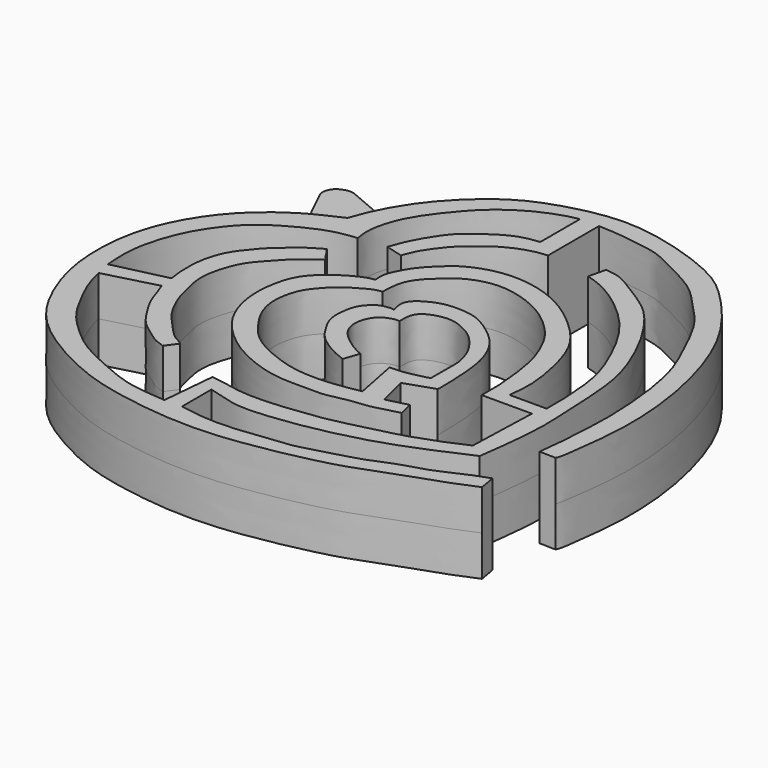
from build123d import *

# Parameters (mm, degrees)
F1_DEPTH    = 3.5
F3_DEPTH    = 2.5
F4_T1_DEPTH = 9.423215052
F4_T3_DEPTH = 7.2035331062
F4_T5_DEPTH = 6.3861082138
F6_R        = 1.3203003793
F7_DEPTH    = 5


# Not quite as in the source:
# - a fillet or chamfer that OpenCascade refuses, or shapes differently, is made with other operations: its cross-section is extruded or revolved along the edge and cut away or added
# - the dataset's text gives a spline's control points without its knots; the knots are read off the source's solid


with BuildPart() as f1:
    # F0 (on Top) → F1 (new body, symmetric)
    with BuildSketch(Plane.XY):
        with BuildLine():
            add(Edge.make_bspline(
                [(62.0494894683, 22.5223191082), (61.5763515234, 22.534451137), (61.1032135785, 22.5465831657), (60.6300756335, 22.5587151945)],
                knots=[0, 0, 0, 0, 1.4198803856, 1.4198803856, 1.4198803856, 1.4198803856], degree=3))
            add(Edge.make_bspline(
                [(29.0716737509, 41.1939695477), (29.306027893, 41.857310813), (29.8115589063, 43.2882259688), (31.339767814, 45.8344011789), (33.0379336105, 47.8185700655), (35.9160335187, 50.4486482505), (40.2057484134, 52.0426798575), (45.48861495, 52.9328004198), (52.9165185764, 50.5280179099), (55.6796708405, 48.398356233), (59.724609742, 43.8025024951), (61.9112576233, 37.8696812405), (62.8091572498, 32.726443865), (62.9266276354, 28.2018625321), (62.4240936499, 24.4927107006), (62.2361245052, 22.9214412082), (62.0494894683, 22.5223191082)],
                knots=[0, 0, 0, 0, 0.0521380391, 0.111927968, 0.1689619765, 0.2371588921, 0.3113537891, 0.3933259358, 0.4892077049, 0.5553764335, 0.6402636071, 0.729148712, 0.8091940033, 0.8840304935, 0.9524124, 1, 1, 1, 1], degree=3))
            add(Edge.make_bspline(
                [(60.8482062817, 16.0528682172), (60.4288818862, 15.8716763746), (59.534784142, 15.4853386593), (57.7264506978, 14.7998216857), (55.8708508075, 14.2034203061), (52.630731068, 12.9646220618), (50.9585172951, 12.4005941246), (47.9810616659, 11.6593155695), (45.2557239075, 11.174386798), (42.1471963462, 10.6964826332), (38.5794281807, 10.6237297735), (35.038597522, 10.9933372199), (30.8346536369, 11.7868657529), (27.2082918083, 13.3540305822), (23.6378704785, 15.5218973851), (21.3228934365, 17.9769063359), (19.6730407733, 21.3203975306), (18.6287885283, 25.130340922), (18.7791180909, 31.25108759), (22.1258241288, 36.9758945902), (26.2799285315, 39.9800364052), (27.8457582196, 40.6097996518), (29.0716737509, 41.1939695477)],
                knots=[0, 0, 0, 0, 0.0323172073, 0.0693227416, 0.1082559513, 0.158008347, 0.1950607871, 0.2415647298, 0.2872565248, 0.3350937464, 0.3860886927, 0.4374690356, 0.4931770933, 0.5474283537, 0.602365058, 0.6518805178, 0.7032339004, 0.7568993464, 0.8230773105, 0.8928533254, 0.9519441527, 1, 1, 1, 1], degree=3))
            add(Edge.make_bspline(
                [(60.5880208313, 17.5061523914), (60.6747493148, 17.0217243334), (60.7614777982, 16.5372962753), (60.8482062817, 16.0528682172)],
                knots=[0, 0, 0, 0, 1.4763913301, 1.4763913301, 1.4763913301, 1.4763913301], degree=3))
            add(Edge.make_bspline(
                [(37.5935249031, 12.5934553022), (38.0452848145, 12.531038319), (39.3071128132, 12.2668629621), (42.2147455771, 12.1754331807), (44.8674374333, 12.6506329659), (46.9396252013, 12.6974842254), (49.4646264533, 13.5274050404), (51.9887441448, 14.1045960088), (54.493210959, 15.2813445301), (56.3991158532, 15.6585487305), (59.124650253, 17.0151377844), (59.7854045823, 17.2054630189), (60.5880208313, 17.5061523914)],
                knots=[0, 0, 0, 0, 0.0839677582, 0.1958350575, 0.3028773071, 0.3959940813, 0.5007707763, 0.6070837185, 0.7133171176, 0.8066213923, 0.9144743817, 1, 1, 1, 1], degree=3))
            add(Edge.make_bspline(
                [(37.5935249031, 15.7923810184), (37.5935249031, 14.7863343979), (37.5935249031, 13.5995019227), (37.5935249031, 12.5934553022)],
                knots=[0, 0, 0, 0, 3.1989257162, 3.1989257162, 3.1989257162, 3.1989257162], degree=3))
            add(Edge.make_bspline(
                [(57.8698590398, 19.5260569453), (57.2722614614, 19.2518359716), (55.9374419677, 18.6547629093), (52.8317063751, 17.3486047041), (49.8839991865, 16.3833590419), (46.0118602733, 15.4908640908), (42.551168035, 15.058897568), (40.0725237694, 14.9739274299), (38.4607709731, 15.5945353022), (37.5935249031, 15.7923810184)],
                knots=[0, 0, 0, 0, 0.1197639567, 0.270468062, 0.4182518209, 0.5834884644, 0.7385810257, 0.8671389586, 1, 1, 1, 1], degree=3))
            add(Edge.make_bspline(
                [(47.4926754832, 46.1788736284), (47.927789971, 46.1352208019), (48.8780404031, 46.0398870027), (50.4485854452, 45.005540302), (52.793619445, 43.6144483568), (54.3147090185, 41.8964903618), (55.7547999729, 39.6954989953), (56.982321959, 37.1233650238), (57.9331963192, 34.4453501838), (58.2647103385, 31.2739474412), (58.3992190946, 27.6715420395), (58.5145376309, 25.6548387921), (58.3120615211, 22.7856589167), (58.0217878255, 20.6459678244), (57.8698590398, 19.5260569453)],
                knots=[0, 0, 0, 0, 0.0597690308, 0.1305301224, 0.2161422502, 0.2947520123, 0.3783962884, 0.4660421153, 0.5528551466, 0.6465286275, 0.7443886958, 0.8183602325, 0.9049300376, 1, 1, 1, 1], degree=3))
            add(Edge.make_bspline(
                [(47.1493708197, 44.6869616846), (47.2638057075, 45.1842656659), (47.3782405954, 45.6815696471), (47.4926754832, 46.1788736284)],
                knots=[0, 0, 0, 0, 1.5309014795, 1.5309014795, 1.5309014795, 1.5309014795], degree=3))
            add(Edge.make_bspline(
                [(57.0660457015, 27.7780741453), (57.0828094684, 28.3480911337), (57.0833657213, 29.4686732532), (56.9658779649, 31.452071832), (56.6597337165, 33.9116675307), (55.5444065948, 36.7282621966), (53.6693378682, 40.3548979754), (50.6815931716, 43.0058324291), (48.6285551485, 44.2222707419), (47.6501277942, 44.5268467146), (47.1493708197, 44.6869616846)],
                knots=[0, 0, 0, 0, 0.1014033342, 0.2110947118, 0.3333142833, 0.4693488673, 0.6282984434, 0.7850184408, 0.9039004269, 1, 1, 1, 1], degree=3))
            add(Edge.make_bspline(
                [(53.8438558578, 27.7780741453), (54.9179191391, 27.7780741453), (55.9919824203, 27.7780741453), (57.0660457015, 27.7780741453)],
                knots=[0, 0, 0, 0, 3.2221898437, 3.2221898437, 3.2221898437, 3.2221898437], degree=3))
            add(Edge.make_bspline(
                [(36.206882447, 35.2931544185), (36.1764845234, 35.5885803582), (36.1091925015, 36.2385932325), (36.6806068453, 37.4538685554), (37.3234322074, 38.5065184037), (38.5682458967, 39.7628057228), (39.7512814872, 40.7306689733), (42.5740597709, 41.7085320293), (45.9900359962, 41.2527105843), (48.8118848265, 39.8512735993), (51.2771955701, 37.6919484665), (52.6516823052, 35.8494727467), (53.4784180909, 33.5058638977), (53.9772231874, 30.8429033195), (54.0206694547, 29.2081760616), (53.9057321855, 28.3065811845), (53.8438558578, 27.7780741453)],
                knots=[0, 0, 0, 0, 0.0478150567, 0.1043645776, 0.1606219176, 0.225642618, 0.2873527464, 0.3715879872, 0.4636992782, 0.552438077, 0.6418664152, 0.7167824888, 0.7952255164, 0.8774223597, 0.9403869977, 1, 1, 1, 1], degree=3))
            add(Edge.make_bspline(
                [(49.791354686, 21.1576391011), (49.3382530631, 21.0376215345), (48.4902822396, 20.8130148085), (47.4767508433, 20.5043809637), (45.7231368878, 20.4183214673), (43.9634570973, 19.9068264066), (42.4944829734, 20.0241891308), (39.8604343147, 19.887922666), (37.1297080189, 20.7597202692), (35.0182532448, 21.8681586876), (32.9047601837, 23.6604882614), (31.6103804887, 25.6766069916), (30.9739740641, 28.0749194036), (31.1244725286, 30.4733894793), (31.7519799581, 32.5781705802), (33.5391654159, 34.172439048), (35.1990013305, 35.0808547127), (35.8615062461, 35.257202768), (36.206882447, 35.2931544185)],
                knots=[0, 0, 0, 0, 0.0512751396, 0.0967288377, 0.1552682074, 0.2149058996, 0.2683746399, 0.3397682684, 0.4148452727, 0.4835069411, 0.5564865603, 0.6248731942, 0.6939737689, 0.7623566152, 0.8270847949, 0.8952845577, 0.9556608186, 1, 1, 1, 1], degree=3))
            add(Edge.make_bspline(
                [(49.4943931699, 22.4225744605), (49.5933803419, 22.0009293407), (49.692367514, 21.5792842209), (49.791354686, 21.1576391011)],
                knots=[0, 0, 0, 0, 1.2993258273, 1.2993258273, 1.2993258273, 1.2993258273], degree=3))
            add(Edge.make_bspline(
                [(47.6537831128, 21.9598766416), (48.2673197985, 22.1141092479), (48.8808564842, 22.2683418542), (49.4943931699, 22.4225744605)],
                knots=[0, 0, 0, 0, 1.8978763537, 1.8978763537, 1.8978763537, 1.8978763537], degree=3))
            add(Edge.make_bspline(
                [(46.9948574901, 24.5558936149), (47.2144993643, 23.6905546238), (47.4341412385, 22.8252156327), (47.6537831128, 21.9598766416)],
                knots=[0, 0, 0, 0, 2.6783366296, 2.6783366296, 2.6783366296, 2.6783366296], degree=3))
            add(Edge.make_bspline(
                [(49.4943931699, 25.4038851708), (48.6612146099, 25.1212213188), (47.82803605, 24.8385574669), (46.9948574901, 24.5558936149)],
                knots=[0, 0, 0, 0, 2.6394636375, 2.6394636375, 2.6394636375, 2.6394636375], degree=3))
            add(Edge.make_bspline(
                [(39.9363972247, 32.6340422034), (39.8842838138, 32.8398562354), (39.7825802868, 33.2412074209), (39.7317090705, 33.8407763364), (40.1424327532, 34.4939511839), (40.9435667079, 34.98708908), (41.8689153893, 35.4022832836), (43.0578273832, 35.5288732917), (44.5042341477, 35.4172964468), (45.7031414177, 34.9277042276), (47.4978658208, 33.6142505705), (48.5069398345, 32.3164872915), (49.1750692015, 30.6332309556), (49.4127095767, 28.8730099925), (49.4897749365, 27.47010552), (49.5663415678, 25.7261840891), (49.5163608933, 25.5028841557), (49.4943931699, 25.4038851708)],
                knots=[0, 0, 0, 0, 0.0486624325, 0.0951159794, 0.1471567147, 0.20648322, 0.2679859547, 0.3350675936, 0.4079143723, 0.4781740436, 0.5686991634, 0.6479717232, 0.7297791406, 0.8106862151, 0.886747396, 0.9656619823, 1, 1, 1, 1], degree=3))
            add(Edge.make_bspline(
                [(41.731480509, 24.8407628387), (41.440631405, 24.9485887841), (40.8168018985, 25.1798651314), (39.7916131994, 25.7534846132), (38.7559420202, 26.5272756625), (38.0982481114, 27.4898951264), (37.2875541922, 28.8560847254), (37.3574485466, 30.3452179464), (37.6091145936, 31.571109546), (38.568811942, 32.5305731387), (39.2786992519, 32.6748706607), (39.7982324544, 32.7072710049), (39.9363972247, 32.6340422034)],
                knots=[0, 0, 0, 0, 0.0923950748, 0.1949164593, 0.3010659305, 0.4031182199, 0.5202614288, 0.6339443109, 0.739345279, 0.8450787721, 0.9263091339, 1, 1, 1, 1], degree=3))
            add(Edge.make_bspline(
                [(42.1944595873, 26.199799031), (42.0401332279, 25.7467869669), (41.8858068685, 25.2937749028), (41.731480509, 24.8407628387)],
                knots=[0, 0, 0, 0, 1.4357329135, 1.4357329135, 1.4357329135, 1.4357329135], degree=3))
            add(Edge.make_bspline(
                [(41.2784581907, 31.5763664872), (41.1436027927, 31.5858341266), (40.8403638146, 31.6097808209), (40.2362607189, 31.4043893185), (39.5927274842, 30.9978187711), (39.1784076019, 30.1464339224), (39.0659228719, 29.4295308466), (39.2309271665, 28.4702577556), (39.979528122, 27.528420715), (41.1981351902, 26.6654285399), (41.6937363632, 26.4125064221), (42.0679750848, 26.2360667755), (42.1944595873, 26.199799031)],
                knots=[0, 0, 0, 0, 0.0735226239, 0.1624191671, 0.2605026822, 0.3681233171, 0.4640931201, 0.5716419619, 0.6967882033, 0.8336292207, 0.9199382159, 1, 1, 1, 1], degree=3))
            add(Edge.make_bspline(
                [(48.1486208737, 26.3907369226), (48.1407468106, 26.8014264215), (48.1249530554, 28.1574826059), (48.2288835515, 29.260214228), (47.8216074376, 30.7540843594), (47.1971116739, 31.7848959678), (46.435927977, 32.6753941876), (45.7728156443, 33.1898699892), (44.5756440395, 33.8070333041), (43.4669023743, 33.9744272395), (42.0250272432, 33.6085927619), (41.2430052697, 32.8206115327), (41.2670391516, 32.0012648354), (41.2784581907, 31.5763664872)],
                knots=[0, 0, 0, 0, 0.1067685372, 0.1965667749, 0.2958638337, 0.3871372355, 0.4739417602, 0.549517036, 0.6427533045, 0.7302902948, 0.828194732, 0.9103637064, 1, 1, 1, 1], degree=3))
            add(Edge.make_bspline(
                [(44.9851080775, 25.8539021015), (45.4219860375, 25.8806252604), (46.2626284099, 25.8809088613), (47.208258913, 26.1637437155), (47.8616882143, 26.2615828811), (48.1486208737, 26.3907369226)],
                knots=[0, 0, 0, 0, 0.3648118806, 0.6850183006, 1, 1, 1, 1], degree=3))
            add(Edge.make_bspline(
                [(45.7483939826, 21.9598766416), (45.4939653476, 23.2578851283), (45.2395367126, 24.5558936149), (44.9851080775, 25.8539021015)],
                knots=[0, 0, 0, 0, 3.9681279787, 3.9681279787, 3.9681279787, 3.9681279787], degree=3))
            add(Edge.make_bspline(
                [(37.6781485975, 34.2296846211), (37.4404118501, 34.1936868052), (36.9248820688, 34.1220552019), (36.0572276042, 33.5790584889), (34.969351795, 33.007191617), (33.7116272309, 31.6576174543), (33.0250916628, 30.6155309796), (32.5469725534, 28.3648756243), (33.292716879, 26.3648713305), (34.1485984224, 25.1332402542), (35.0683346813, 23.9369652337), (36.4140307347, 22.972945278), (38.1110135143, 22.2170279083), (40.252083112, 21.514821624), (43.1220565262, 21.487846839), (44.8876694045, 21.8039903534), (45.7483939826, 21.9598766416)],
                knots=[0, 0, 0, 0, 0.0470759388, 0.1014443874, 0.162981057, 0.2361593674, 0.2979693267, 0.3790337951, 0.4585299897, 0.5253581662, 0.5918114662, 0.6616615194, 0.735923773, 0.8179351352, 0.9103719411, 1, 1, 1, 1], degree=3))
            add(Edge.make_bspline(
                [(52.3898104827, 26.5814382583), (52.4009236356, 27.1473973257), (52.422608099, 28.3284507078), (52.2339233546, 30.355819257), (51.8418938845, 33.0599256238), (50.7376318904, 35.5392708539), (49.6186905356, 36.9373328644), (47.9253669377, 38.4697088862), (45.4552778952, 39.6147669279), (42.8546664852, 39.989725932), (40.6509516266, 39.1817195979), (39.3514751131, 38.0710048359), (37.7393561929, 36.4275672316), (37.6985092177, 34.9608070194), (37.6781485975, 34.2296846211)],
                knots=[0, 0, 0, 0, 0.07336606, 0.1531121462, 0.2464440072, 0.3380288381, 0.4124441862, 0.495906265, 0.5884062651, 0.6787253687, 0.7622014119, 0.8357701318, 0.9181388862, 1, 1, 1, 1], degree=3))
            add(Edge.make_bspline(
                [(56.7519466082, 26.5814382583), (55.297901233, 26.5814382583), (53.8438558578, 26.5814382583), (52.3898104827, 26.5814382583)],
                knots=[0, 0, 0, 0, 4.3621361256, 4.3621361256, 4.3621361256, 4.3621361256], degree=3))
            add(Edge.make_bspline(
                [(56.5444603562, 20.4251520336), (56.6150570909, 22.4772474418), (56.6813498735, 24.52934285), (56.7519466082, 26.5814382583)],
                knots=[0, 0, 0, 0, 6.1597817027, 6.1597817027, 6.1597817027, 6.1597817027], degree=3))
            add(Edge.make_bspline(
                [(36.4984497428, 17.2690122078), (36.9061818341, 17.1824827732), (37.7624563088, 17.1295248841), (39.0762184566, 16.743449065), (41.659563732, 16.6860947729), (44.0992037425, 16.9754605145), (46.27518064, 17.2270052266), (48.270570816, 17.712679766), (50.4263134482, 18.2642328403), (51.943600097, 18.6174788035), (54.0581224203, 19.3695526663), (55.5057995415, 19.9433434205), (56.0856204092, 20.2797500823), (56.5444603562, 20.4251520336)],
                knots=[0, 0, 0, 0, 0.0745300415, 0.1525667333, 0.2596775198, 0.3663080261, 0.4646849665, 0.5613972858, 0.6602103449, 0.7450811446, 0.8452892234, 0.9278090092, 1, 1, 1, 1], degree=3))
            add(Edge.make_bspline(
                [(36.0700786114, 12.5934553022), (36.2128689885, 14.2126102), (36.3556593657, 15.64985731), (36.4984497428, 17.2690122078)],
                knots=[0, 0, 0, 0, 4.6951394232, 4.6951394232, 4.6951394232, 4.6951394232], degree=3))
            add(Edge.make_bspline(
                [(20.9572687745, 24.3625063449), (20.9901233087, 24.1942706248), (21.0678958144, 23.7943819484), (21.3866486093, 22.7730052466), (21.8410977302, 21.6779831246), (22.5618618858, 20.2858198339), (23.5658316666, 18.4569642539), (25.4701688523, 16.6545082602), (27.0049310002, 15.4059909191), (29.0971823948, 14.3916633668), (31.2755716049, 13.4138173776), (33.3554212502, 12.7702262818), (35.1510001469, 12.679946413), (36.0700786114, 12.5934553022)],
                knots=[0, 0, 0, 0, 0.0506784114, 0.1200859802, 0.1942970801, 0.2783327008, 0.3766915169, 0.4858996024, 0.5814866125, 0.6840659965, 0.788697898, 0.8883454566, 1, 1, 1, 1], degree=3))
            add(Edge.make_bspline(
                [(25.4806894809, 25.5635473877), (23.9278276761, 25.1632003735), (22.5101305793, 24.7628533592), (20.9572687745, 24.3625063449)],
                knots=[0, 0, 0, 0, 4.6801532532, 4.6801532532, 4.6801532532, 4.6801532532], degree=3))
            add(Edge.make_bspline(
                [(31.0146547854, 18.7400026868), (30.77927245, 18.8391094784), (30.1178986731, 18.9887179154), (29.1847780616, 19.748494201), (28.0256959577, 20.5152103853), (27.2156271205, 21.7060226052), (26.1628366252, 23.3866591182), (25.8908202249, 24.5410535619), (25.5849009401, 25.1454231238), (25.4806894809, 25.5635473877)],
                knots=[0, 0, 0, 0, 0.1184724448, 0.2567863776, 0.4034898088, 0.5558748194, 0.7325974378, 0.8679249237, 1, 1, 1, 1], degree=3))
            add(Edge.make_bspline(
                [(31.7300595343, 19.7239623715), (31.4871246616, 19.3885136396), (31.2575896581, 19.0754514188), (31.0146547854, 18.7400026868)],
                knots=[0, 0, 0, 0, 1.2165445393, 1.2165445393, 1.2165445393, 1.2165445393], degree=3))
            add(Edge.make_bspline(
                [(31.7300595343, 35.4503169656), (31.3647890329, 35.2863434192), (30.8443023829, 34.7678790108), (29.7625315594, 33.9901222243), (28.8707593931, 32.9635892933), (27.817315966, 31.847341728), (27.1709175273, 30.4553129635), (26.6285465869, 28.3522887479), (27.0245959038, 26.4701972551), (27.4977202214, 24.6132537143), (28.5097274014, 22.7021276556), (29.5833780815, 21.5670667267), (30.8481802888, 20.1307424145), (31.474123302, 19.9557794886), (31.7300595343, 19.7239623715)],
                knots=[0, 0, 0, 0, 0.070093621, 0.1456206838, 0.2231371095, 0.3040395367, 0.3860403594, 0.4823076234, 0.5735149405, 0.6654806136, 0.7612978726, 0.8459764481, 0.9350349245, 1, 1, 1, 1], degree=3))
            add(Edge.make_bspline(
                [(30.8207478374, 36.760546267), (31.178633372, 36.3238031665), (31.3721739997, 35.8870600661), (31.7300595343, 35.4503169656)],
                knots=[0, 0, 0, 0, 1.5948506464, 1.5948506464, 1.5948506464, 1.5948506464], degree=3))
            add(Edge.make_bspline(
                [(25.2884849906, 26.8364176154), (25.2440446701, 27.1217748051), (25.1487668492, 27.7503889455), (25.0967780301, 28.9966732121), (25.2299385454, 30.4842215591), (25.7742609862, 32.1466596959), (26.8287490269, 33.4966955344), (27.729168979, 34.5208320529), (28.8773117145, 35.4476611522), (29.7686140192, 36.1949823553), (30.5059019143, 36.5604378782), (30.8207478374, 36.760546267)],
                knots=[0, 0, 0, 0, 0.0910260221, 0.1972742163, 0.3144585912, 0.4406924452, 0.5651314103, 0.6774182986, 0.7926321416, 0.8964902037, 1, 1, 1, 1], degree=3))
            add(Edge.make_bspline(
                [(20.6440426409, 25.7492437959), (22.1921900908, 26.1116350691), (23.7403375407, 26.4740263422), (25.2884849906, 26.8364176154)],
                knots=[0, 0, 0, 0, 4.7699886429, 4.7699886429, 4.7699886429, 4.7699886429], degree=3))
            add(Edge.make_bspline(
                [(31.4588211477, 39.2978303134), (31.3789239588, 39.3015193105), (31.158102101, 39.3113269226), (30.2299417942, 39.1746241385), (28.686572436, 38.8162635588), (25.5942646742, 37.2047992743), (23.8165620534, 35.7064927347), (22.1497796262, 33.4206638326), (21.1918876243, 31.2628642636), (20.4387488473, 28.4514696809), (20.581920115, 26.6377320454), (20.6440426409, 25.7492437959)],
                knots=[0, 0, 0, 0, 0.0414118483, 0.1145200109, 0.2154957329, 0.3618238952, 0.4848046339, 0.6147415316, 0.7370166925, 0.8701626205, 1, 1, 1, 1], degree=3))
            add(Edge.make_bspline(
                [(41.4689593017, 50.8962869644), (41.1492624212, 50.8333973968), (40.4003135361, 50.6860452132), (38.7121623399, 50.0509618593), (37.2514338516, 49.2415729792), (35.6483957025, 48.0920003343), (34.2938338369, 46.6122445214), (32.8961653374, 44.8391458209), (31.9546479002, 43.2613157294), (31.3502809123, 41.3813898861), (31.3146860364, 40.088205068), (31.4322323803, 39.4932992971), (31.4588211477, 39.2978303134)],
                knots=[0, 0, 0, 0, 0.0809110442, 0.1855340284, 0.2880591679, 0.3969963197, 0.5088560904, 0.6261125862, 0.7333553341, 0.8428606459, 0.9322584731, 1, 1, 1, 1], degree=3))
            add(Edge.make_bspline(
                [(41.4689593017, 46.5870350599), (41.4689593017, 48.0234523614), (41.4689593017, 49.4598696629), (41.4689593017, 50.8962869644)],
                knots=[0, 0, 0, 0, 4.3092519045, 4.3092519045, 4.3092519045, 4.3092519045], degree=3))
            add(Edge.make_bspline(
                [(33.8251776993, 39.5700521767), (33.9036570625, 39.7694489732), (34.0534392705, 40.2398558504), (34.3632844694, 41.0088776584), (34.8403488546, 41.9290903453), (35.4746350368, 42.942125168), (36.214897024, 43.9383422602), (37.2177987614, 44.7456514037), (38.2836215731, 45.4925792896), (39.561838236, 46.2553443665), (40.8375425002, 46.5384229229), (41.2611352403, 46.5445169876), (41.4689593017, 46.5870350599)],
                knots=[0, 0, 0, 0, 0.0800890937, 0.1678002136, 0.2657852426, 0.3713458539, 0.4785293651, 0.5870236333, 0.6971666798, 0.8158180333, 0.924100839, 1, 1, 1, 1], degree=3))
            add(Edge.make_bspline(
                [(35.3241302073, 39.1637347639), (34.8244793713, 39.2991739015), (34.3248285353, 39.4346130391), (33.8251776993, 39.5700521767)],
                knots=[0, 0, 0, 0, 1.5530461877, 1.5530461877, 1.5530461877, 1.5530461877], degree=3))
            add(Edge.make_bspline(
                [(43.1099198759, 45.3760661185), (42.7632561839, 45.3486142711), (42.084386205, 45.2843633217), (40.7250786974, 44.853909813), (39.3639222003, 44.1399114417), (38.1326994528, 43.109943656), (37.0935350696, 42.2263032758), (36.2341536196, 41.0331678682), (35.6167644476, 40.049675035), (35.4496204073, 39.4468230997), (35.3241302073, 39.1637347639)],
                knots=[0, 0, 0, 0, 0.1108302146, 0.2404342533, 0.3774853776, 0.5158865681, 0.6445322299, 0.7772164593, 0.8949660251, 1, 1, 1, 1], degree=3))
            add(Edge.make_bspline(
                [(43.1099198759, 50.8962869644), (43.1099198759, 49.0562133491), (43.1099198759, 47.2161397338), (43.1099198759, 45.3760661185)],
                knots=[0, 0, 0, 0, 5.5202208459, 5.5202208459, 5.5202208459, 5.5202208459], degree=3))
            add(Edge.make_bspline(
                [(60.6300756335, 22.5587151945), (60.6755314071, 22.9118751853), (60.7744829602, 23.6806604654), (60.9172479395, 25.2596638586), (60.9798807136, 26.4890204227), (61.0724541444, 28.0959644716), (61.1191718832, 29.6659537847), (60.9952329479, 32.3578816377), (60.6788019814, 35.0128802547), (60.1853331627, 37.3045339858), (59.5407463411, 38.9654022513), (58.29688975, 41.6787817009), (56.9992934358, 44.0950407956), (55.1457914393, 45.9366091789), (53.559412718, 47.755915439), (50.9358648616, 49.0697457013), (48.803106748, 50.214898465), (46.9274731026, 50.5374150264), (44.9334594305, 50.8182479009), (43.7085109185, 50.8706700348), (43.1099198759, 50.8962869644)],
                knots=[0, 0, 0, 0, 0.0408445927, 0.0889135873, 0.1321931947, 0.17999171, 0.2284777408, 0.2912963161, 0.3553036955, 0.4131621764, 0.4644812794, 0.5304639079, 0.5948032383, 0.6561944698, 0.7157607879, 0.7814051217, 0.8411602255, 0.8937562905, 0.9480822808, 1, 1, 1, 1], degree=3))
        make_face()
    extrude(amount=F1_DEPTH, both=True)

    # F2 (on Top) → F3 (join, symmetric)
    with BuildSketch(Plane.XY):
        with BuildLine():
            add(Edge.make_bspline(
                [(30.2500113872, 43.9528679265), (30.1197446268, 43.7145093001), (29.6169976623, 42.7375166644), (29.306027893, 41.857310813), (29.0716737509, 41.1939695477)],
                knots=[0.9311492006, 0.9311492006, 0.9311492006, 0.9311492006, 0.9478619609, 1, 1, 1, 1], degree=3))
            Line((30.2500113872, 43.9528679265), (25.6518474154, 45.9167640379))
            Line((25.6518474154, 45.9167640379), (24.1825316626, 45.4618074086))
            Line((24.1825316626, 45.4618074086), (24.1825316626, 44.3714354442))
            Line((24.1825316626, 44.3714354442), (26.375665907, 39.8780890105))
            add(Edge.make_bspline(
                [(29.0716737509, 41.1939695477), (27.903743968, 40.6374308611), (27.2110827748, 40.3547424964), (26.375665907, 39.8780890105)],
                knots=[0, 0, 0, 0, 0.045782808, 0.045782808, 0.045782808, 0.045782808], degree=3))
        make_face()
    extrude(amount=F3_DEPTH, both=True)

    # F4: fillet of radius 1.2 on 3 edges, made by hand

    # F4_s2 → F4_t1 (cut)
    with BuildSketch(Plane.XY.offset(-4.711607526)):
        with BuildLine():
            ThreePointArc((24.1825316626, 44.5771643982), (24.4166309288, 45.2892288422), (25.0275912834, 45.7234703465))
            Line((25.0275912834, 45.7234703465), (24.1825316626, 45.4618074086))
            Line((24.1825316626, 45.4618074086), (24.1825316626, 44.5771643982))
        make_face()
    extrude(amount=F4_T1_DEPTH, mode=Mode.SUBTRACT)

    # F4_s4 → F4_t3 (cut)
    with BuildSketch(Plane.XY.offset(-3.6017665531)):
        with BuildLine():
            ThreePointArc((26.0571356782, 45.7436636334), (25.6477985833, 45.8385016447), (25.2308602309, 45.7864102252))
            Line((25.2308602309, 45.7864102252), (25.6518474154, 45.9167640379))
            Line((25.6518474154, 45.9167640379), (26.0571356782, 45.7436636334))
        make_face()
    extrude(amount=F4_T3_DEPTH, mode=Mode.SUBTRACT)

    # F4_s6 → F4_t5 (cut)
    with BuildSketch(Plane.XY.offset(-3.1930541069)):
        with BuildLine():
            ThreePointArc((24.3041285182, 44.1223048682), (24.2133259978, 44.378549491), (24.1825316626, 44.648657087))
            Line((24.1825316626, 44.648657087), (24.1825316626, 44.3714354442))
            Line((24.1825316626, 44.3714354442), (24.3041285182, 44.1223048682))
        make_face()
    extrude(amount=F4_T5_DEPTH, mode=Mode.SUBTRACT)

    # F6 (on 3pt) → F7 (cut, symmetric)
    with BuildSketch(Plane(origin=(31.3091565551, 39.4167106584, 0), x_dir=(-0.7830368213, 0.6219753504, 0), z_dir=(0.6219753504, 0.7830368213, 0))):
        with Locations((6.4161866903, 0)):
            Circle(F6_R)
    extrude(amount=F7_DEPTH, both=True, mode=Mode.SUBTRACT)


solid = f1.part
